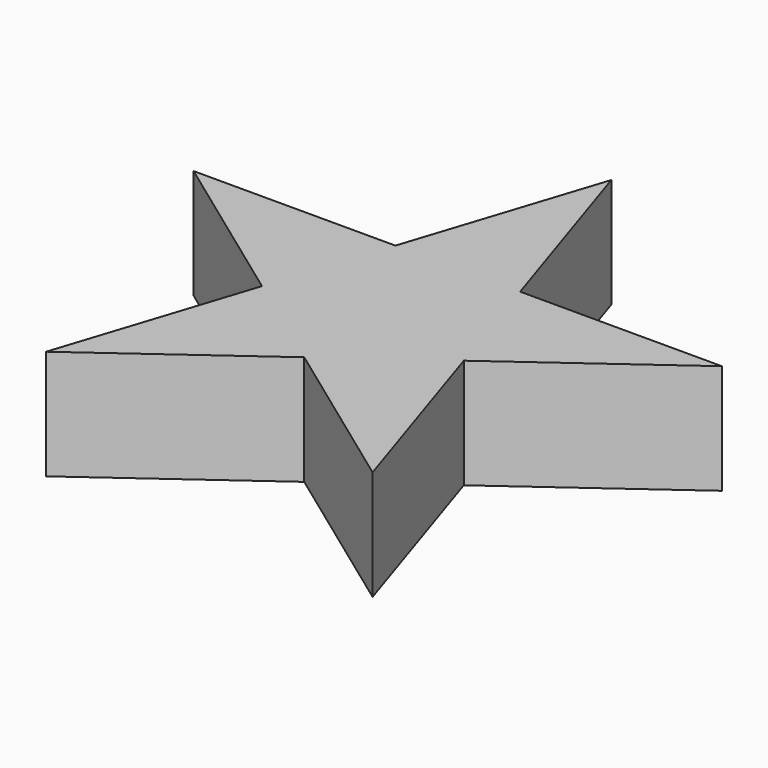
from build123d import *

# Parameters (mm, degrees)
F1_DEPTH = 0.4
F5_DEPTH = 12.7
F6_DEPTH = 12.7


with BuildPart() as f1:
    # F0 (on Top) → F1 (new body)
    with BuildSketch(Plane.XY):
        Polygon((-31.5438667271, -25.7632551613), (-12.0486849532, -39.9273338113), (-19.495181774, -62.8452944863), (0, -48.6812158363), (19.495181774, -62.8452944863), (12.0486849532, -39.9273338113), (31.5438667271, -25.7632551613), (7.4464968208, -25.7632551613), (0, -2.8452944863), (-7.4464968208, -25.7632551613), align=None)
    extrude(amount=F1_DEPTH)

    # F2 (on face) → F5 (join)
    with BuildSketch(Plane.XY.offset(0.4)):
        Polygon((9.747590887, -32.8452944863), (7.4464968208, -25.7632551613), (0, -2.8452944863), (-7.4464968208, -25.7632551613), (-31.5438667271, -25.7632551613), (-12.0486849532, -39.9273338113), (-19.495181774, -62.8452944863), (0, -48.6812158363), (19.495181774, -62.8452944863), (12.0486849532, -39.9273338113), align=None)
        Polygon((31.5438667271, -25.7632551613), (9.747590887, -32.8452944863), (12.0486849532, -39.9273338113), align=None)
    extrude(amount=F5_DEPTH)

    # F6 (add): a face of the model
    f6_faces = [f1.faces().sort_by_distance(p)[0] for p in [
        (16.2459848116, -28.1239349363, 0.4),
    ]]
    extrude(f6_faces, amount=F6_DEPTH)


solid = f1.part
